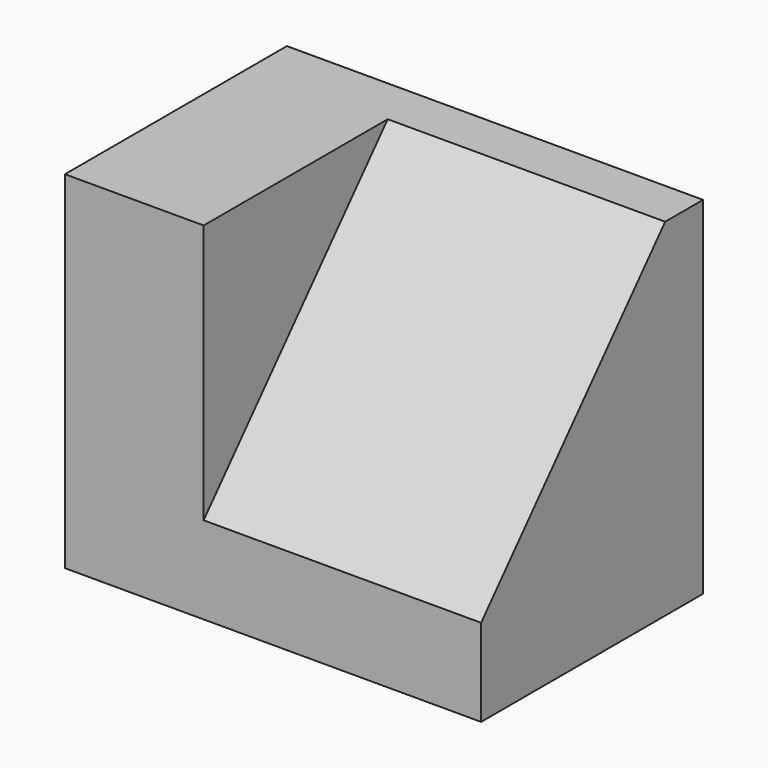
from build123d import *

# Parameters (mm, degrees)
F0_W     = 38.1
F0_H     = 31.75
F1_DEPTH = 25.4
F4_DEPTH = 25.4


# Not quite as in the source:
# - a feature of the source that left no trace in its solid (it failed there, or was rolled back) is left out


with BuildPart() as f1:
    # F0 (on Front) → F1 (new body)
    with BuildSketch(Plane.XZ):
        with Locations((-31.4665150195, 15.875)):
            Rectangle(F0_W, F0_H)
    extrude(amount=F1_DEPTH)

    # F2 (on face) → F4 (cut)
    with BuildSketch(Plane.YZ.offset(-12.4165150195)):
        Polygon((-25.4, 7.9906463393), (-4.3392399561, 31.75), (-25.4, 31.75), align=None)
    extrude(amount=-F4_DEPTH, mode=Mode.SUBTRACT)


solid = f1.part
